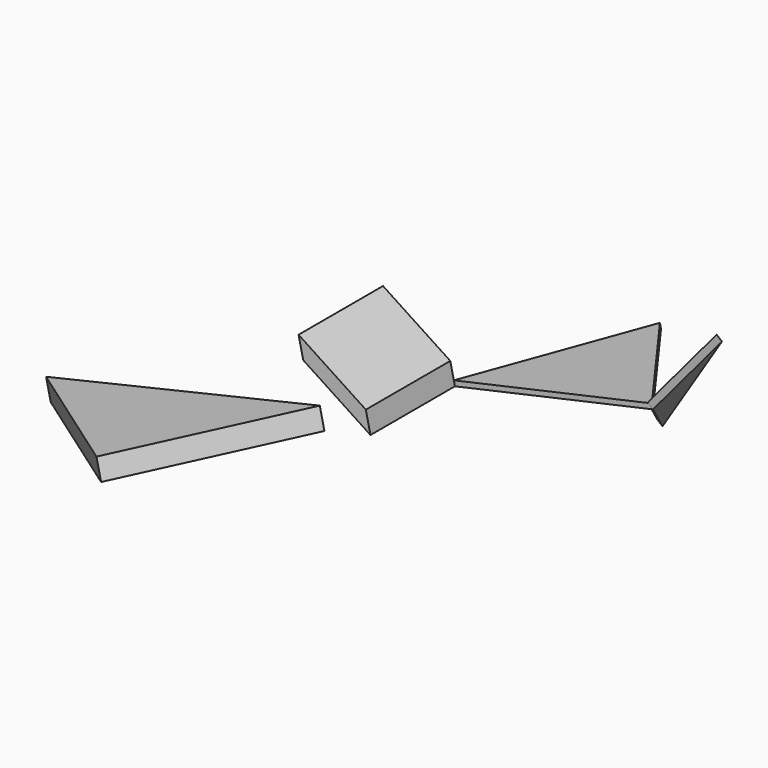
from build123d import *

# Parameters (mm, degrees)
F1_E6_W  = 32.5085211131
F1_E6_H  = 42.672
F3_DEPTH = 8.636
F5_DEPTH = 2.032
F7_DEPTH = 2.794


with BuildPart() as f3:
    # F2 (on face) + F1_E6 (on explicit) → F3 (new body)
    with BuildSketch(Plane(origin=(17.2792129444, 0, -77.6114316477), x_dir=(0.9761011501, 0, 0.2173166925), z_dir=(-0.2173166925, 0, 0.9761011501))):
        Polygon((0, -43.6379054688), (-111.5465760231, -45.830283314), (-46.496912837, -99.7414588928), align=None)
    with BuildSketch(Plane(origin=(35.1171717048, 0, -73.6400336027), x_dir=(-0.8363188208, 0, 0.548243404), z_dir=(0.548243404, 0, 0.8363188208))):
        with Locations((16.2542605566, 21.336)):
            Rectangle(F1_E6_W, F1_E6_H)
    extrude(amount=F3_DEPTH, dir=(-0.2173166925, 0, 0.9761011501))


with BuildPart() as f5:
    # F4 (on face) → F5 (new body)
    with BuildSketch(Plane(origin=(17.2792129444, 0, -77.6114316477), x_dir=(0.9761011501, 0, 0.2173166925), z_dir=(-0.2173166925, 0, 0.9761011501))):
        Polygon((54.9373701215, 59.3950413167), (18.2747031485, 0), (100.2867293219, 0), align=None)
    extrude(amount=F5_DEPTH)

    # F6 (on face) → F7 (join)
    with BuildSketch(Plane(origin=(94.1781769889, 0, -80.4043797496), x_dir=(0, -1, 0), z_dir=(-0.7605311042, 0, 0.6493015013))):
        Polygon((1.9783186726, 77.6898695076), (-34.3080833554, -4.0362984873), (0, 32.3286296737), align=None)
    extrude(amount=F7_DEPTH)


solid = Compound([f3.part, f5.part])
